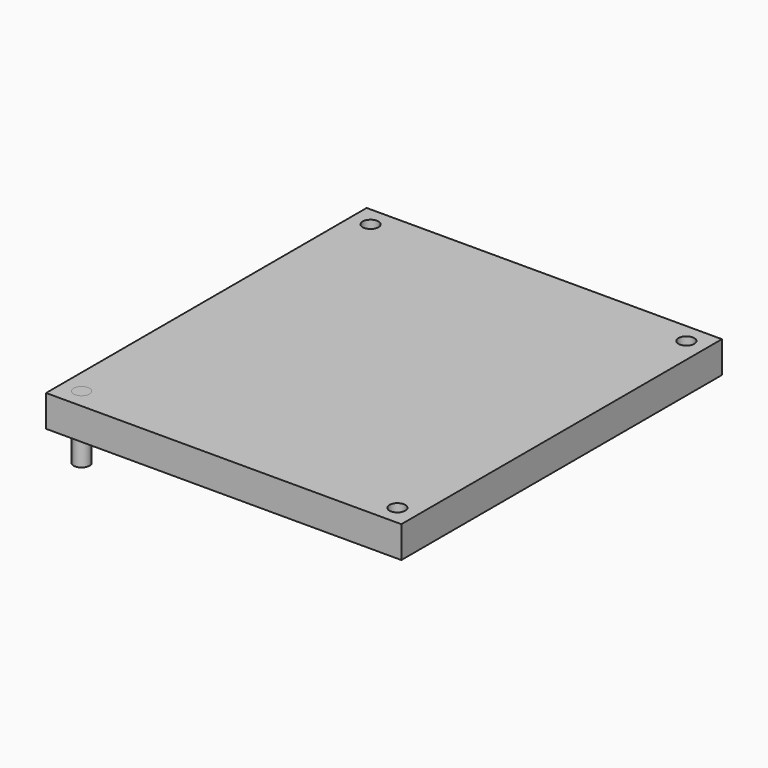
from build123d import *

# Parameters (mm, degrees)
F0_W     = 450
F0_H     = 507.5829336092
F0_R     = 10
F1_DEPTH = 40
F2_R     = 10
F3_DEPTH = 80


# Not quite as in the source:
# - the program builds the solid bodies; features that only make, move or delete a surface that nothing else refers to are left out


with BuildPart() as f1:
    # F0 (on Top) → F1 (new body)
    with BuildSketch(Plane.XY):
        Rectangle(F0_W, F0_H)
        with Locations((-200, -228.7914668046)):
            Circle(F0_R, mode=Mode.SUBTRACT)
        with Locations((200, -228.7914668046)):
            Circle(F0_R, mode=Mode.SUBTRACT)
        with Locations((-200, 228.7914668046)):
            Circle(F0_R, mode=Mode.SUBTRACT)
        with Locations((200, 228.7914668046)):
            Circle(F0_R, mode=Mode.SUBTRACT)
    extrude(amount=F1_DEPTH)


with BuildPart() as f3:
    # F2 (on face) → F3 (new body)
    with BuildSketch(Plane.XY.offset(40)):
        with Locations((-200, -228.7914668046)):
            Circle(F2_R)
    extrude(amount=-F3_DEPTH)


solid = Compound([f1.part, f3.part])
